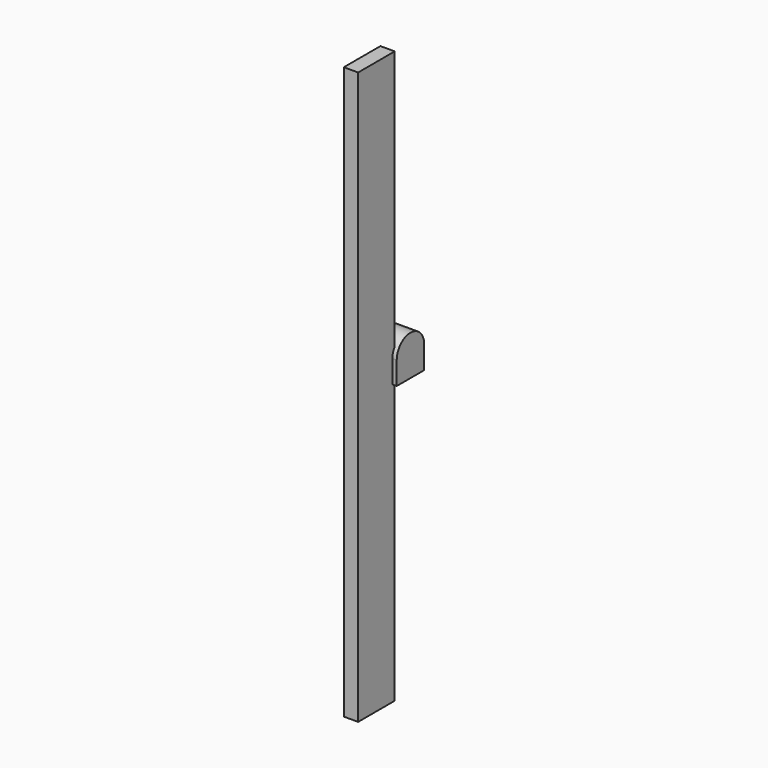
from build123d import *

# Parameters (mm, degrees)
F1_DEPTH = 2.5
F2_DEPTH = 4


# Not quite as in the source:
# - a feature names something its author has since deleted; it is built from what else it names


with BuildPart() as f1:
    # F0 (on Right) → F1 (new body, symmetric)
    with BuildSketch(Plane.YZ):
        with BuildLine():
            Line((-11, 102.1741141677), (-27, 102.1741141677))
            Line((-27, 102.1741141677), (-27, -97.8258858323))
            Line((-27, -97.8258858323), (-11, -97.8258858323))
            Line((-11, -97.8258858323), (-11, 0))
            Line((-11, 0), (-12, 0))
            Line((-12, 0), (-12, 8))
            ThreePointArc((-12, 8), (-11.7445626465, 9.7320508076), (-11, 11.3166247904))
            Line((-11, 11.3166247904), (-11, 102.1741141677))
        make_face()
        with BuildLine():
            Line((-11, 0), (-11, 11.3166247904))
            ThreePointArc((-11, 11.3166247904), (-11.7445626465, 9.7320508076), (-12, 8))
            Line((-12, 8), (-12, 0))
            Line((-12, 0), (-11, 0))
        make_face()
    extrude(amount=F1_DEPTH, both=True)

    # F0 (on Right) → F2 (join, symmetric)
    with BuildSketch(Plane.YZ):
        with BuildLine():
            ThreePointArc((0, 8), (-4.2679491924, 13.7445626465), (-11, 11.3166247904))
            Line((-11, 11.3166247904), (-11, 0))
            Line((-11, 0), (0, 0))
            Line((0, 0), (0, 8))
        make_face()
        with BuildLine():
            Line((-11, 0), (-11, 11.3166247904))
            ThreePointArc((-11, 11.3166247904), (-11.7445626465, 9.7320508076), (-12, 8))
            Line((-12, 8), (-12, 0))
            Line((-12, 0), (-11, 0))
        make_face()
    extrude(amount=F2_DEPTH, both=True)


solid = f1.part
